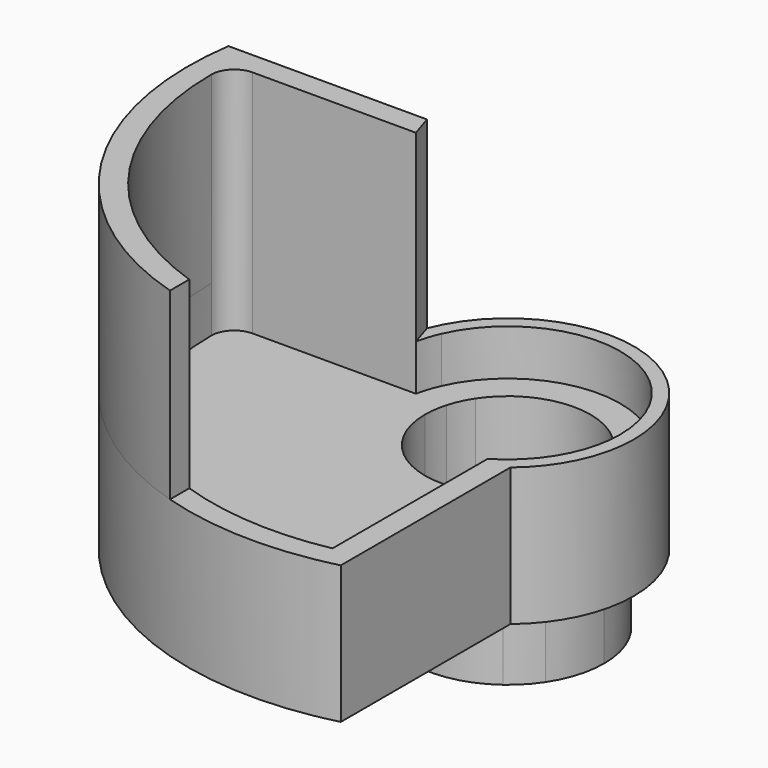
from build123d import *

# Parameters (mm, degrees)
F1_DEPTH    = 2
F2_DEPTH    = 3
F3_DEPTH    = 1.5
F5_DEPTH    = 4
F6_T1_DEPTH = 6.2509414233


# Not quite as in the source:
# - a fillet or chamfer that OpenCascade refuses, or shapes differently, is made with other operations: its cross-section is extruded or revolved along the edge and cut away or added
# - a feature names something its author has since deleted; it is built from what else it names


with BuildPart() as f1:
    # F0 (on Top) → F1 (new body)
    with BuildSketch(Plane.XY):
        with BuildLine():
            ThreePointArc((-2.398436991, 0.5), (-2.3309771289, 0.7543511281), (-2.2366269246, 1))
            Line((-2.2366269246, 1), (-2.556369496, 1))
            ThreePointArc((-2.556369496, 1), (-2.6395896521, 0.7533866658), (-2.6990785465, 0.5))
            Line((-2.6990785465, 0.5), (-2.398436991, 0.5))
        make_face()
        with BuildLine():
            ThreePointArc((-2.2366269246, 1), (0.5112553348, 2.3960630173), (2.45, 0))
            ThreePointArc((2.45, 0), (2.2682592444, -0.9260129589), (1.75, -1.7146428199))
            Line((1.75, -1.7146428199), (1.75, -2.1148345089))
            ThreePointArc((1.75, -2.1148345089), (2.483825175, -1.1686049375), (2.745, 0))
            ThreePointArc((2.745, 0), (0.5088176164, 2.6974301906), (-2.556369496, 1))
            Line((-2.556369496, 1), (-2.2366269246, 1))
        make_face()
        with BuildLine():
            ThreePointArc((-2.6990785465, 0.5), (-2.6395896521, 0.7533866658), (-2.556369496, 1))
            Line((-2.556369496, 1), (-6.3720091023, 1))
            ThreePointArc((-6.3720091023, 1), (-6.4061799882, 0.7505717543), (-6.4305909526, 0.5))
            Line((-6.4305909526, 0.5), (-2.6990785465, 0.5))
        make_face()
        with BuildLine():
            ThreePointArc((-2.745, 0), (-2.7334955286, 0.2510521758), (-2.6990785465, 0.5))
            Line((-2.6990785465, 0.5), (-6.4305909526, 0.5))
            ThreePointArc((-6.4305909526, 0.5), (-6.4451459116, 0.2501882847), (-6.45, 0))
            Line((-6.45, 0), (-2.745, 0))
        make_face()
        with BuildLine():
            Line((1.25, -6.3277168078), (1.25, -2.4438749968))
            ThreePointArc((1.25, -2.4438749968), (-1.4324410983, -2.341610023), (-2.745, 0))
            Line((-2.745, 0), (-6.45, 0))
            ThreePointArc((-6.45, 0), (-4.0951190459, -4.9832218494), (1.25, -6.3277168078))
        make_face()
        with BuildLine():
            Line((1.25, -2.4438749968), (1.25, -2.1071307506))
            ThreePointArc((1.25, -2.1071307506), (-1.2124355653, -2.1289668856), (-2.45, 0))
            Line((-2.45, 0), (-2.745, 0))
            ThreePointArc((-2.745, 0), (-1.4324410983, -2.341610023), (1.25, -2.4438749968))
        make_face()
        with BuildLine():
            Line((1.75, -2.1148345089), (1.75, -1.7146428199))
            ThreePointArc((1.75, -1.7146428199), (1.5127827649, -1.927171063), (1.25, -2.1071307506))
            Line((1.25, -2.1071307506), (1.25, -2.4438749968))
            ThreePointArc((1.25, -2.4438749968), (1.5089953316, -2.2930237873), (1.75, -2.1148345089))
        make_face()
        with BuildLine():
            Line((1.75, -6.2080592781), (1.75, -2.1148345089))
            ThreePointArc((1.75, -2.1148345089), (1.5089953316, -2.2930237873), (1.25, -2.4438749968))
            Line((1.25, -2.4438749968), (1.25, -6.3277168078))
            ThreePointArc((1.25, -6.3277168078), (1.5011926862, -6.272871792), (1.75, -6.2080592781))
        make_face()
        with BuildLine():
            ThreePointArc((-6.4305909526, 0.5), (-6.4061799882, 0.7505717543), (-6.3720091023, 1))
            Line((-6.3720091023, 1), (-6.8776812953, 1))
            ThreePointArc((-6.8776812953, 1), (-6.9093605068, 0.7504914307), (-6.931991056, 0.5))
            Line((-6.931991056, 0.5), (-6.4305909526, 0.5))
        make_face()
        with BuildLine():
            Line((1.75, -6.7260686883), (1.75, -6.2080592781))
            ThreePointArc((1.75, -6.2080592781), (1.5011926862, -6.272871792), (1.25, -6.3277168078))
            Line((1.25, -6.3277168078), (1.25, -6.8366658541))
            ThreePointArc((1.25, -6.8366658541), (1.501018965, -6.7859739218), (1.75, -6.7260686883))
        make_face()
        with BuildLine():
            Line((1.25, -6.8366658541), (1.25, -6.3277168078))
            ThreePointArc((1.25, -6.3277168078), (-4.0951190459, -4.9832218494), (-6.45, 0))
            Line((-6.45, 0), (-6.95, 0))
            ThreePointArc((-6.95, 0), (-4.4505617623, -5.3380708126), (1.25, -6.8366658541))
        make_face()
        with BuildLine():
            ThreePointArc((-6.45, 0), (-6.4451459116, 0.2501882847), (-6.4305909526, 0.5))
            Line((-6.4305909526, 0.5), (-6.931991056, 0.5))
            ThreePointArc((-6.931991056, 0.5), (-6.9454963048, 0.2501621085), (-6.95, 0))
            Line((-6.95, 0), (-6.45, 0))
        make_face()
        with BuildLine():
            ThreePointArc((-2.45, 0), (-2.4370751556, 0.2513258562), (-2.398436991, 0.5))
            Line((-2.398436991, 0.5), (-2.6990785465, 0.5))
            ThreePointArc((-2.6990785465, 0.5), (-2.7334955286, 0.2510521758), (-2.745, 0))
            Line((-2.745, 0), (-2.45, 0))
        make_face()
        with BuildLine():
            ThreePointArc((-2.45, 0), (-1.2124355653, -2.1289668856), (1.25, -2.1071307506))
            Line((1.25, -2.1071307506), (1.25, -1.6874537031))
            ThreePointArc((1.25, -1.6874537031), (-0.9447221814, -1.8754999334), (-2.1, 0))
            Line((-2.1, 0), (-2.45, 0))
        make_face()
        with BuildLine():
            ThreePointArc((-2.1, 0), (-0.9447221814, -1.8754999334), (1.25, -1.6874537031))
            Line((1.25, -1.6874537031), (1.25, -1.2951833847))
            ThreePointArc((1.25, -1.2951833847), (-0.703562364, -1.6568041526), (-1.8, 0))
            Line((-1.8, 0), (-2.1, 0))
        make_face()
        with BuildLine():
            Line((-2.0396078054, 0.5), (-2.398436991, 0.5))
            ThreePointArc((-2.398436991, 0.5), (-2.4370751556, 0.2513258562), (-2.45, 0))
            Line((-2.45, 0), (-2.1, 0))
            ThreePointArc((-2.1, 0), (-2.0848472835, 0.2518170056), (-2.0396078054, 0.5))
        make_face()
        with BuildLine():
            Line((-1.8466185313, 1), (-2.2366269246, 1))
            ThreePointArc((-2.2366269246, 1), (-2.3309771289, 0.7543511281), (-2.398436991, 0.5))
            Line((-2.398436991, 0.5), (-2.0396078054, 0.5))
            ThreePointArc((-2.0396078054, 0.5), (-1.9591295988, 0.7561819986), (-1.8466185313, 1))
        make_face()
        with BuildLine():
            Line((2.1, 0), (2.45, 0))
            ThreePointArc((2.45, 0), (0.5112553348, 2.3960630173), (-2.2366269246, 1))
            Line((-2.2366269246, 1), (-1.8466185313, 1))
            ThreePointArc((-1.8466185313, 1), (0.5158008745, 2.0356692899), (2.1, 0))
        make_face()
        with BuildLine():
            Line((-1.7291616466, 0.5), (-2.0396078054, 0.5))
            ThreePointArc((-2.0396078054, 0.5), (-2.0848472835, 0.2518170056), (-2.1, 0))
            Line((-2.1, 0), (-1.8, 0))
            ThreePointArc((-1.8, 0), (-1.7822024245, 0.2524965704), (-1.7291616466, 0.5))
        make_face()
        with BuildLine():
            Line((-1.4966629547, 1), (-1.8466185313, 1))
            ThreePointArc((-1.8466185313, 1), (-1.9591295988, 0.7561819986), (-2.0396078054, 0.5))
            Line((-2.0396078054, 0.5), (-1.7291616466, 0.5))
            ThreePointArc((-1.7291616466, 0.5), (-1.6321721997, 0.7589558027), (-1.4966629547, 1))
        make_face()
        with BuildLine():
            Line((1.8, 0), (2.1, 0))
            ThreePointArc((2.1, 0), (0.5158008745, 2.0356692899), (-1.8466185313, 1))
            Line((-1.8466185313, 1), (-1.4966629547, 1))
            ThreePointArc((-1.4966629547, 1), (0.522497216, 1.722497216), (1.8, 0))
        make_face()
        with BuildLine():
            ThreePointArc((1.25, -1.6874537031), (1.5229366739, -1.4459128214), (1.75, -1.1608186766))
            Line((1.75, -1.1608186766), (1.75, -0.4213074887))
            ThreePointArc((1.75, -0.4213074887), (1.5623427186, -0.8939156725), (1.25, -1.2951833847))
            Line((1.25, -1.2951833847), (1.25, -1.6874537031))
        make_face()
        with BuildLine():
            ThreePointArc((1.25, -2.1071307506), (1.5127827649, -1.927171063), (1.75, -1.7146428199))
            Line((1.75, -1.7146428199), (1.75, -1.1608186766))
            ThreePointArc((1.75, -1.1608186766), (1.5229366739, -1.4459128214), (1.25, -1.6874537031))
            Line((1.25, -1.6874537031), (1.25, -2.1071307506))
        make_face()
        with BuildLine():
            ThreePointArc((1.75, -1.1608186766), (2.0105969263, -0.6062177826), (2.1, 0))
            Line((2.1, 0), (1.8, 0))
            ThreePointArc((1.8, 0), (1.7874562932, -0.2121320344), (1.75, -0.4213074887))
            Line((1.75, -0.4213074887), (1.75, -1.1608186766))
        make_face()
        with BuildLine():
            ThreePointArc((1.75, -1.7146428199), (2.2682592444, -0.9260129589), (2.45, 0))
            Line((2.45, 0), (2.1, 0))
            ThreePointArc((2.1, 0), (2.0105969263, -0.6062177826), (1.75, -1.1608186766))
            Line((1.75, -1.1608186766), (1.75, -1.7146428199))
        make_face()
    extrude(amount=F1_DEPTH)

    # F0 (on Top) → F2 (join)
    with BuildSketch(Plane.XY):
        with BuildLine():
            ThreePointArc((-6.4305909526, 0.5), (-6.4061799882, 0.7505717543), (-6.3720091023, 1))
            Line((-6.3720091023, 1), (-6.8776812953, 1))
            ThreePointArc((-6.8776812953, 1), (-6.9093605068, 0.7504914307), (-6.931991056, 0.5))
            Line((-6.931991056, 0.5), (-6.4305909526, 0.5))
        make_face()
        with BuildLine():
            ThreePointArc((-2.6990785465, 0.5), (-2.6395896521, 0.7533866658), (-2.556369496, 1))
            Line((-2.556369496, 1), (-6.3720091023, 1))
            ThreePointArc((-6.3720091023, 1), (-6.4061799882, 0.7505717543), (-6.4305909526, 0.5))
            Line((-6.4305909526, 0.5), (-2.6990785465, 0.5))
        make_face()
        with BuildLine():
            ThreePointArc((-2.398436991, 0.5), (-2.3309771289, 0.7543511281), (-2.2366269246, 1))
            Line((-2.2366269246, 1), (-2.556369496, 1))
            ThreePointArc((-2.556369496, 1), (-2.6395896521, 0.7533866658), (-2.6990785465, 0.5))
            Line((-2.6990785465, 0.5), (-2.398436991, 0.5))
        make_face()
        with BuildLine():
            ThreePointArc((-2.2366269246, 1), (0.5112553348, 2.3960630173), (2.45, 0))
            ThreePointArc((2.45, 0), (2.2682592444, -0.9260129589), (1.75, -1.7146428199))
            Line((1.75, -1.7146428199), (1.75, -2.1148345089))
            ThreePointArc((1.75, -2.1148345089), (2.483825175, -1.1686049375), (2.745, 0))
            ThreePointArc((2.745, 0), (0.5088176164, 2.6974301906), (-2.556369496, 1))
            Line((-2.556369496, 1), (-2.2366269246, 1))
        make_face()
        with BuildLine():
            Line((1.75, -2.1148345089), (1.75, -1.7146428199))
            ThreePointArc((1.75, -1.7146428199), (1.5127827649, -1.927171063), (1.25, -2.1071307506))
            Line((1.25, -2.1071307506), (1.25, -2.4438749968))
            ThreePointArc((1.25, -2.4438749968), (1.5089953316, -2.2930237873), (1.75, -2.1148345089))
        make_face()
        with BuildLine():
            Line((1.75, -6.2080592781), (1.75, -2.1148345089))
            ThreePointArc((1.75, -2.1148345089), (1.5089953316, -2.2930237873), (1.25, -2.4438749968))
            Line((1.25, -2.4438749968), (1.25, -6.3277168078))
            ThreePointArc((1.25, -6.3277168078), (1.5011926862, -6.272871792), (1.75, -6.2080592781))
        make_face()
        with BuildLine():
            Line((1.75, -6.7260686883), (1.75, -6.2080592781))
            ThreePointArc((1.75, -6.2080592781), (1.5011926862, -6.272871792), (1.25, -6.3277168078))
            Line((1.25, -6.3277168078), (1.25, -6.8366658541))
            ThreePointArc((1.25, -6.8366658541), (1.501018965, -6.7859739218), (1.75, -6.7260686883))
        make_face()
        with BuildLine():
            Line((1.25, -6.8366658541), (1.25, -6.3277168078))
            ThreePointArc((1.25, -6.3277168078), (-4.0951190459, -4.9832218494), (-6.45, 0))
            Line((-6.45, 0), (-6.95, 0))
            ThreePointArc((-6.95, 0), (-4.4505617623, -5.3380708126), (1.25, -6.8366658541))
        make_face()
        with BuildLine():
            ThreePointArc((-6.45, 0), (-6.4451459116, 0.2501882847), (-6.4305909526, 0.5))
            Line((-6.4305909526, 0.5), (-6.931991056, 0.5))
            ThreePointArc((-6.931991056, 0.5), (-6.9454963048, 0.2501621085), (-6.95, 0))
            Line((-6.95, 0), (-6.45, 0))
        make_face()
    extrude(amount=F2_DEPTH)

    # F0 (on Top) → F3 (join)
    with BuildSketch(Plane.XY):
        with BuildLine():
            Line((1.8, 0), (2.1, 0))
            ThreePointArc((2.1, 0), (0.5158008745, 2.0356692899), (-1.8466185313, 1))
            Line((-1.8466185313, 1), (-1.4966629547, 1))
            ThreePointArc((-1.4966629547, 1), (0.522497216, 1.722497216), (1.8, 0))
        make_face()
        with BuildLine():
            Line((-1.4966629547, 1), (-1.8466185313, 1))
            ThreePointArc((-1.8466185313, 1), (-1.9591295988, 0.7561819986), (-2.0396078054, 0.5))
            Line((-2.0396078054, 0.5), (-1.7291616466, 0.5))
            ThreePointArc((-1.7291616466, 0.5), (-1.6321721997, 0.7589558027), (-1.4966629547, 1))
        make_face()
        with BuildLine():
            Line((-1.7291616466, 0.5), (-2.0396078054, 0.5))
            ThreePointArc((-2.0396078054, 0.5), (-2.0848472835, 0.2518170056), (-2.1, 0))
            Line((-2.1, 0), (-1.8, 0))
            ThreePointArc((-1.8, 0), (-1.7822024245, 0.2524965704), (-1.7291616466, 0.5))
        make_face()
        with BuildLine():
            ThreePointArc((-2.1, 0), (-0.9447221814, -1.8754999334), (1.25, -1.6874537031))
            Line((1.25, -1.6874537031), (1.25, -1.2951833847))
            ThreePointArc((1.25, -1.2951833847), (-0.703562364, -1.6568041526), (-1.8, 0))
            Line((-1.8, 0), (-2.1, 0))
        make_face()
        with BuildLine():
            ThreePointArc((1.25, -1.6874537031), (1.5229366739, -1.4459128214), (1.75, -1.1608186766))
            Line((1.75, -1.1608186766), (1.75, -0.4213074887))
            ThreePointArc((1.75, -0.4213074887), (1.5623427186, -0.8939156725), (1.25, -1.2951833847))
            Line((1.25, -1.2951833847), (1.25, -1.6874537031))
        make_face()
        with BuildLine():
            ThreePointArc((1.75, -1.1608186766), (2.0105969263, -0.6062177826), (2.1, 0))
            Line((2.1, 0), (1.8, 0))
            ThreePointArc((1.8, 0), (1.7874562932, -0.2121320344), (1.75, -0.4213074887))
            Line((1.75, -0.4213074887), (1.75, -1.1608186766))
        make_face()
    extrude(amount=-F3_DEPTH)

    # F4 (on face) → F5 (join)
    with BuildSketch(Plane.XY.offset(3)):
        with BuildLine():
            Line((-2.398436991, 0.5), (-2.556369496, 1))
            Line((-2.556369496, 1), (-6.8776812953, 1))
            ThreePointArc((-6.8776812953, 1), (-5.8706460858, -3.7199481898), (-2.0327166243, -6.6460938246))
            Line((-2.0327166243, -6.6460938246), (-2.0327166243, -6.1213203743))
            ThreePointArc((-2.0327166243, -6.1213203743), (-5.3728358118, -3.5686321385), (-6.4305909526, 0.5))
            Line((-6.4305909526, 0.5), (-2.398436991, 0.5))
        make_face()
    extrude(amount=F5_DEPTH)

    # F6: fillet of radius 0.5 on 1 edges, made by hand

    # F6_s2 → F6_t1 (join)
    with BuildSketch(Plane.XY.offset(0.7490585767)):
        with BuildLine():
            ThreePointArc((-5.95, 0.5), (-6.3035533906, 0.3535533906), (-6.45, 0))
            ThreePointArc((-6.45, 0), (-6.4451459116, 0.2501882847), (-6.4305909526, 0.5))
            Line((-6.4305909526, 0.5), (-5.95, 0.5))
        make_face()
    extrude(amount=F6_T1_DEPTH)


solid = f1.part
